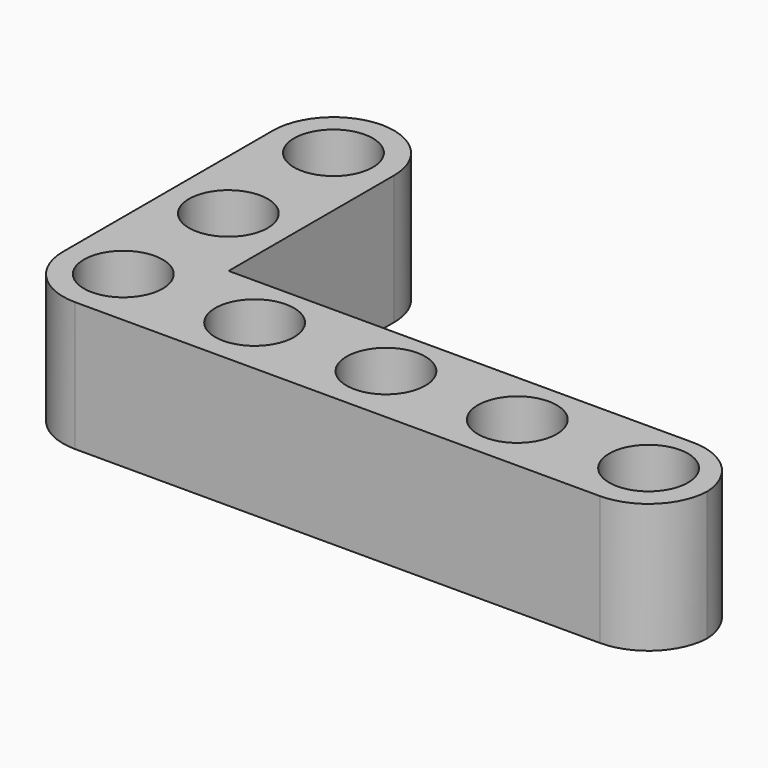
from build123d import *

# Parameters (mm, degrees)
F0_R        = 2.4
F1_DEPTH    = 7.88
F2_T1_DEPTH = 26.405


# Not quite as in the source:
# - a fillet or chamfer that OpenCascade refuses, or shapes differently, is made with other operations: its cross-section is extruded or revolved along the edge and cut away or added


with BuildPart() as f1:
    # F0 (on Top) → F1 (new body)
    with BuildSketch(Plane.XY):
        Polygon((-48.3995083171, -5.7841986276), (-31.3221290569, -5.7841986276), (-9.0295083171, -5.7841986276), (-9.0295083171, 1.2940158032), (-41.0095083171, 1.2940158032), (-41.0095083171, 17.5958013724), (-48.3995083171, 17.5958013724), align=None)
        with Locations((-44.7195083171, -2.0891986276)):
            Circle(F0_R, mode=Mode.SUBTRACT)
        with Locations((-36.7195083171, -2.0891986276)):
            Circle(F0_R, mode=Mode.SUBTRACT)
        with BuildLine():
            ThreePointArc((-28.7195083171, -4.4891986276), (-31.1195083171, -2.0891986276), (-28.7195083171, 0.3108013724))
            ThreePointArc((-28.7195083171, 0.3108013724), (-26.3195083171, -2.0891986276), (-28.7195083171, -4.4891986276))
        make_face(mode=Mode.SUBTRACT)
        with BuildLine():
            ThreePointArc((-20.7195083171, -4.4891986276), (-23.1195083171, -2.0891986276), (-20.7195083171, 0.3108013724))
            ThreePointArc((-20.7195083171, 0.3108013724), (-18.3195083171, -2.0891986276), (-20.7195083171, -4.4891986276))
        make_face(mode=Mode.SUBTRACT)
        with BuildLine():
            ThreePointArc((-12.7195083171, -4.4891986276), (-15.1195083171, -2.0891986276), (-12.7195083171, 0.3108013724))
            ThreePointArc((-12.7195083171, 0.3108013724), (-10.3195083171, -2.0891986276), (-12.7195083171, -4.4891986276))
        make_face(mode=Mode.SUBTRACT)
        with Locations((-44.7195083171, 5.9108013724)):
            Circle(F0_R, mode=Mode.SUBTRACT)
        with Locations((-44.7195083171, 13.9108013724)):
            Circle(F0_R, mode=Mode.SUBTRACT)
    extrude(amount=F1_DEPTH)

    # F2: fillet of radius 3.705 on 5 edges, made by hand

    # F2_s2 → F2_t1 (cut)
    with BuildSketch(Plane.XY.offset(-9.2625)):
        with BuildLine():
            ThreePointArc((-48.3995083171, 13.8908013724), (-47.3143389413, 16.5106319967), (-44.6945083171, 17.5958013724))
            Line((-44.6945083171, 17.5958013724), (-48.3995083171, 17.5958013724))
            Line((-48.3995083171, 17.5958013724), (-48.3995083171, 13.8908013724))
        make_face()
        with BuildLine():
            ThreePointArc((-41.0095083171, 13.8908013724), (-42.0946776928, 16.5106319967), (-44.7145083171, 17.5958013724))
            Line((-44.7145083171, 17.5958013724), (-41.0095083171, 17.5958013724))
            Line((-41.0095083171, 17.5958013724), (-41.0095083171, 13.8908013724))
        make_face()
        with BuildLine():
            ThreePointArc((-9.0295083171, -2.4109841968), (-10.1146776928, 0.2088464274), (-12.7345083171, 1.2940158032))
            Line((-12.7345083171, 1.2940158032), (-9.0295083171, 1.2940158032))
            Line((-9.0295083171, 1.2940158032), (-9.0295083171, -2.4109841968))
        make_face()
        with BuildLine():
            ThreePointArc((-9.0295083171, -2.0791986276), (-10.1146776928, -4.6990292519), (-12.7345083171, -5.7841986276))
            Line((-12.7345083171, -5.7841986276), (-9.0295083171, -5.7841986276))
            Line((-9.0295083171, -5.7841986276), (-9.0295083171, -2.0791986276))
        make_face()
        with BuildLine():
            ThreePointArc((-44.6945083171, -5.7841986276), (-47.3143389413, -4.6990292519), (-48.3995083171, -2.0791986276))
            Line((-48.3995083171, -2.0791986276), (-48.3995083171, -5.7841986276))
            Line((-48.3995083171, -5.7841986276), (-44.6945083171, -5.7841986276))
        make_face()
    extrude(amount=F2_T1_DEPTH, mode=Mode.SUBTRACT)


solid = f1.part
